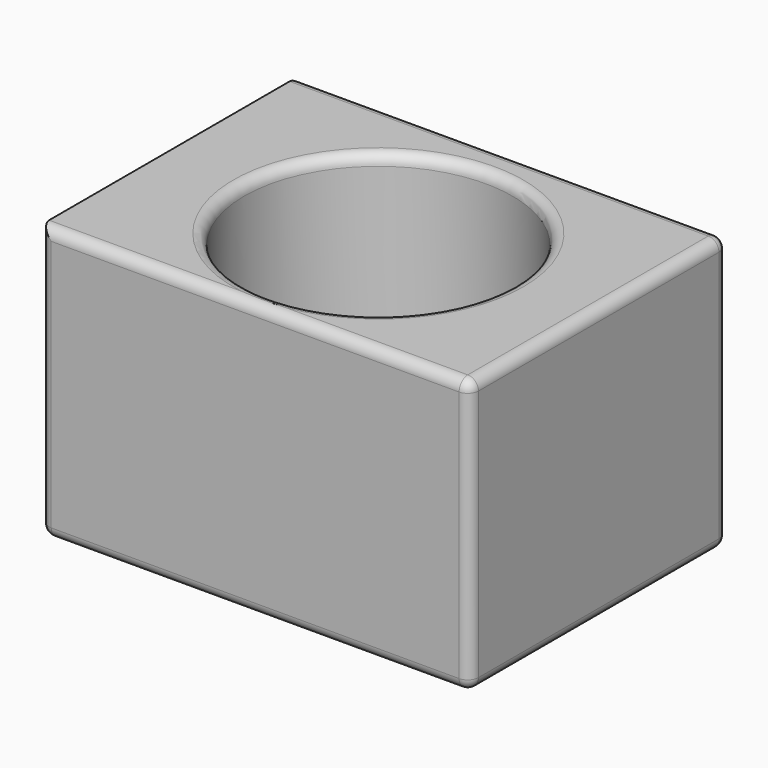
from build123d import *

# Parameters (mm, degrees)
F1_W         = 203.2
F1_H         = 127
F2_DEPTH     = 76.2
F3_D         = 127
F3_DEPTH     = 76.2
F3_TIP       = 38.1546493083
F4_DEPTH     = 2.54
F5_T3_DEPTH  = 210.82
F5_T5_DEPTH  = 142.24
F5_T7_DEPTH  = 193.04
F5_T9_DEPTH  = 137.16
F5_T11_DEPTH = 119.38
F5_S15_W     = 5.08
F5_S15_H     = 5.08
F5_T16_DEPTH = 5.08
F5_S21_W     = 5.08
F5_S21_H     = 5.08
F5_T22_DEPTH = 5.08
F5_S27_W     = 5.08
F5_S27_H     = 5.08
F5_T28_DEPTH = 5.08
F5_S33_W     = 5.08
F5_S33_H     = 5.08
F5_T34_DEPTH = 5.08
F5_S39_W     = 5.08
F5_S39_H     = 5.08
F5_T40_DEPTH = 5.08
F5_S45_W     = 5.08
F5_S45_H     = 5.08
F5_T46_DEPTH = 5.08


# Not quite as in the source:
# - a fillet or chamfer that OpenCascade refuses, or shapes differently, is made with other operations: its cross-section is extruded or revolved along the edge and cut away or added


with BuildPart() as f2:
    # F1 (on Front) → F2 (new body, symmetric)
    with BuildSketch(Plane.XZ):
        with Locations((0, -63.5)):
            Rectangle(F1_W, F1_H)
    extrude(amount=F2_DEPTH, both=True)

    # F3
    with Locations(Plane.XY):
        with Locations((0, -3.3519673161)):
            Hole(F3_D / 2, depth=F3_DEPTH)
            with Locations((0, 0, -(F3_DEPTH + F3_TIP / 2))):  # 118° drill point
                Cone(0, F3_D / 2, F3_TIP, mode=Mode.SUBTRACT)

    # F4 (add): a face of the model
    f4_faces = [f2.faces().sort_by_distance(p)[0] for p in [
        (0, 0, -127),
    ]]
    extrude(f4_faces, amount=F4_DEPTH)

    # F5: fillet of radius 5.08 on 13 edges, made by hand

    # F5_s1 → F5_t2 (revolve)
    with BuildSketch(Plane.XZ.offset(3.3519673161)):
        with BuildLine():
            ThreePointArc((63.5, -73.3258742868), (62.8414069354, -75.8273859721), (61.0363934205, -77.6802841744))
            Line((61.0363934205, -77.6802841744), (63.5, -76.2))
            Line((63.5, -76.2), (63.5, -73.3258742868))
        make_face()
    revolve(axis=Axis((0, -3.3519673161, -76.2), (0, 0, 1)))

    # F5_s4 → F5_t3 (cut)
    with BuildSketch(Plane.YZ.offset(-114.3)):
        with BuildLine():
            ThreePointArc((71.12, 0), (74.7121024484, -1.4878975516), (76.2, -5.08))
            Line((76.2, -5.08), (76.2, 0))
            Line((76.2, 0), (71.12, 0))
        make_face()
        with BuildLine():
            ThreePointArc((-71.12, 0), (-74.7121024484, -1.4878975516), (-76.2, -5.08))
            Line((-76.2, -5.08), (-76.2, 0))
            Line((-76.2, 0), (-71.12, 0))
        make_face()
    extrude(amount=F5_T3_DEPTH, mode=Mode.SUBTRACT)

    # F5_s6 → F5_t5 (cut)
    with BuildSketch(Plane.XZ.offset(-71.12)):
        with BuildLine():
            ThreePointArc((101.6, -5.08), (100.1121024484, -1.4878975516), (96.52, 0))
            Line((96.52, 0), (101.6, 0))
            Line((101.6, 0), (101.6, -5.08))
        make_face()
        with BuildLine():
            ThreePointArc((101.6, -124.46), (100.1121024484, -128.0521024484), (96.52, -129.54))
            Line((96.52, -129.54), (101.6, -129.54))
            Line((101.6, -129.54), (101.6, -124.46))
        make_face()
        with BuildLine():
            ThreePointArc((-96.52, -129.54), (-100.1121024484, -128.0521024484), (-101.6, -124.46))
            Line((-101.6, -124.46), (-101.6, -129.54))
            Line((-101.6, -129.54), (-96.52, -129.54))
        make_face()
    extrude(amount=F5_T5_DEPTH, mode=Mode.SUBTRACT)

    # F5_s8 → F5_t7 (cut)
    with BuildSketch(Plane.YZ.offset(-96.52)):
        with BuildLine():
            ThreePointArc((-76.2, -124.46), (-74.7121024484, -128.0521024484), (-71.12, -129.54))
            Line((-71.12, -129.54), (-76.2, -129.54))
            Line((-76.2, -129.54), (-76.2, -124.46))
        make_face()
        with BuildLine():
            ThreePointArc((71.12, -129.54), (74.7121024484, -128.0521024484), (76.2, -124.46))
            Line((76.2, -124.46), (76.2, -129.54))
            Line((76.2, -129.54), (71.12, -129.54))
        make_face()
    extrude(amount=F5_T7_DEPTH, mode=Mode.SUBTRACT)

    # F5_s10 → F5_t9 (cut)
    with BuildSketch(Plane.XY.offset(-124.46)):
        with BuildLine():
            ThreePointArc((-96.52, -76.2), (-100.1121024484, -74.7121024484), (-101.6, -71.12))
            Line((-101.6, -71.12), (-101.6, -76.2))
            Line((-101.6, -76.2), (-96.52, -76.2))
        make_face()
        with BuildLine():
            ThreePointArc((-96.52, 76.2), (-100.1121024484, 74.7121024484), (-101.6, 71.12))
            Line((-101.6, 71.12), (-101.6, 76.2))
            Line((-101.6, 76.2), (-96.52, 76.2))
        make_face()
    extrude(amount=F5_T9_DEPTH, mode=Mode.SUBTRACT)

    # F5_s12 → F5_t11 (cut)
    with BuildSketch(Plane.XY.offset(-124.46)):
        with BuildLine():
            ThreePointArc((101.6, -71.12), (100.1121024484, -74.7121024484), (96.52, -76.2))
            Line((96.52, -76.2), (101.6, -76.2))
            Line((101.6, -76.2), (101.6, -71.12))
        make_face()
        with BuildLine():
            ThreePointArc((101.6, 71.12), (100.1121024484, 74.7121024484), (96.52, 76.2))
            Line((96.52, 76.2), (101.6, 76.2))
            Line((101.6, 76.2), (101.6, 71.12))
        make_face()
    extrude(amount=F5_T11_DEPTH, mode=Mode.SUBTRACT)


with BuildPart() as f5_tool14:
    # F5_s15 → F5_t16 (new body)
    with BuildSketch(Plane.YZ.offset(96.52)):
        with Locations((73.66, -2.54)):
            Rectangle(F5_S15_W, F5_S15_H)
    extrude(amount=F5_T16_DEPTH)

    # F5_s17 → F5_t18 (revolve, cut)
    with BuildSketch(Plane(origin=(96.52, 71.12, -5.08), x_dir=(0, -0.7071067812, -0.7071067812), z_dir=(0, -0.7071067812, 0.7071067812))):
        with BuildLine():
            ThreePointArc((0, -5.08), (5.08, 0), (0, 5.08))
            Line((0, 5.08), (0, -5.08))
        make_face()
    revolve(axis=Axis((96.52, 71.12, -5.08), (1, 0, 0)), mode=Mode.SUBTRACT)


with BuildPart() as f2_1:
    add(f2.part)

    # F5_t13: cut F5_tool14
    add(f5_tool14.part, mode=Mode.SUBTRACT)


with BuildPart() as f5_tool20:
    # F5_s21 → F5_t22 (new body)
    with BuildSketch(Plane.YZ.offset(96.52)):
        with Locations((-73.66, -2.54)):
            Rectangle(F5_S21_W, F5_S21_H)
    extrude(amount=F5_T22_DEPTH)

    # F5_s23 → F5_t24 (revolve, cut)
    with BuildSketch(Plane(origin=(96.52, -71.12, -5.08), x_dir=(0, 0.7071067812, -0.7071067812), z_dir=(0, -0.7071067812, -0.7071067812))):
        with BuildLine():
            ThreePointArc((0, -5.08), (5.08, 0), (0, 5.08))
            Line((0, 5.08), (0, -5.08))
        make_face()
    revolve(axis=Axis((96.52, -71.12, -5.08), (1, 0, 0)), mode=Mode.SUBTRACT)


with BuildPart() as f2_2:
    add(f2_1.part)

    # F5_t19: cut F5_tool20
    add(f5_tool20.part, mode=Mode.SUBTRACT)


with BuildPart() as f5_tool26:
    # F5_s27 → F5_t28 (new body)
    with BuildSketch(Plane.YZ.offset(96.52)):
        with Locations((-73.66, -127)):
            Rectangle(F5_S27_W, F5_S27_H)
    extrude(amount=F5_T28_DEPTH)

    # F5_s29 → F5_t30 (revolve, cut)
    with BuildSketch(Plane(origin=(96.52, -71.12, -124.46), x_dir=(0, 0.7071067812, 0.7071067812), z_dir=(0, 0.7071067812, -0.7071067812))):
        with BuildLine():
            ThreePointArc((0, -5.08), (5.08, 0), (0, 5.08))
            Line((0, 5.08), (0, -5.08))
        make_face()
    revolve(axis=Axis((96.52, -71.12, -124.46), (1, 0, 0)), mode=Mode.SUBTRACT)


with BuildPart() as f2_3:
    add(f2_2.part)

    # F5_t25: cut F5_tool26
    add(f5_tool26.part, mode=Mode.SUBTRACT)


with BuildPart() as f5_tool32:
    # F5_s33 → F5_t34 (new body)
    with BuildSketch(Plane.YZ.offset(96.52)):
        with Locations((73.66, -127)):
            Rectangle(F5_S33_W, F5_S33_H)
    extrude(amount=F5_T34_DEPTH)

    # F5_s35 → F5_t36 (revolve, cut)
    with BuildSketch(Plane(origin=(96.52, 71.12, -124.46), x_dir=(0, -0.7071067812, 0.7071067812), z_dir=(0, 0.7071067812, 0.7071067812))):
        with BuildLine():
            ThreePointArc((0, -5.08), (5.08, 0), (0, 5.08))
            Line((0, 5.08), (0, -5.08))
        make_face()
    revolve(axis=Axis((96.52, 71.12, -124.46), (1, 0, 0)), mode=Mode.SUBTRACT)


with BuildPart() as f2_4:
    add(f2_3.part)

    # F5_t31: cut F5_tool32
    add(f5_tool32.part, mode=Mode.SUBTRACT)


with BuildPart() as f5_tool38:
    # F5_s39 → F5_t40 (new body)
    with BuildSketch(Plane.XZ.offset(71.12)):
        with Locations((-99.06, -127)):
            Rectangle(F5_S39_W, F5_S39_H)
    extrude(amount=F5_T40_DEPTH)

    # F5_s41 → F5_t42 (revolve, cut)
    with BuildSketch(Plane(origin=(-96.52, -71.12, -124.46), x_dir=(0.7071067812, 0, 0.7071067812), z_dir=(0.7071067812, 0, -0.7071067812))):
        with BuildLine():
            ThreePointArc((0, -5.08), (5.08, 0), (0, 5.08))
            Line((0, 5.08), (0, -5.08))
        make_face()
    revolve(axis=Axis((-96.52, -71.12, -124.46), (0, -1, 0)), mode=Mode.SUBTRACT)


with BuildPart() as f2_5:
    add(f2_4.part)

    # F5_t37: cut F5_tool38
    add(f5_tool38.part, mode=Mode.SUBTRACT)


with BuildPart() as f5_tool44:
    # F5_s45 → F5_t46 (new body)
    with BuildSketch(Plane.XY.offset(-124.46)):
        with Locations((-99.06, 73.66)):
            Rectangle(F5_S45_W, F5_S45_H)
    extrude(amount=-F5_T46_DEPTH)

    # F5_s47 → F5_t48 (revolve, cut)
    with BuildSketch(Plane(origin=(-96.52, 71.12, -124.46), x_dir=(0.7071067812, -0.7071067812, 0), z_dir=(0.7071067812, 0.7071067812, 0))):
        with BuildLine():
            ThreePointArc((0, -5.08), (5.08, 0), (0, 5.08))
            Line((0, 5.08), (0, -5.08))
        make_face()
    revolve(axis=Axis((-96.52, 71.12, -124.46), (0, 0, -1)), mode=Mode.SUBTRACT)


with BuildPart() as f2_6:
    add(f2_5.part)

    # F5_t43: cut F5_tool44
    add(f5_tool44.part, mode=Mode.SUBTRACT)

    # F5_s49 → F5_t50 (revolve, cut)
    with BuildSketch(Plane.XZ.offset(3.3519673161)):
        with BuildLine():
            ThreePointArc((68.58, 0), (64.9878975516, -1.4878975516), (63.5, -5.08))
            Line((63.5, -5.08), (63.5, 0))
            Line((63.5, 0), (68.58, 0))
        make_face()
    revolve(axis=Axis((0, -3.3519673161, 0), (0, 0, 1)), mode=Mode.SUBTRACT)


solid = f2_6.part
